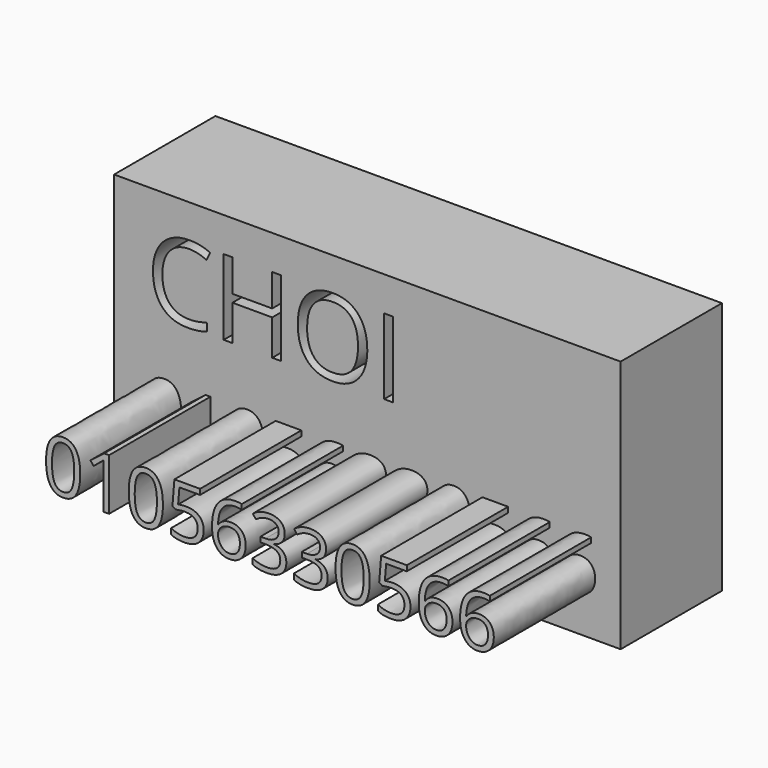
from build123d import *

# Parameters (mm, degrees)
F0_W         = 20
F0_H         = 10
F1_DEPTH     = 5
F2_TEXT_SIZE = 4.1780911346
F3_DEPTH     = 25
F4_TEXT_SIZE = 2.8558414973
F5_DEPTH     = 5


# Not quite as in the source:
# - Text() gives the source's letters only with a copy of the font that has no kerning and outlines rounded to 1/6400 em; it was checked with that copy


with BuildPart() as f1:
    # F0 (on Front) → F1 (new body)
    with BuildSketch(Plane.XZ):
        with Locations((10, 5)):
            Rectangle(F0_W, F0_H)
    extrude(amount=F1_DEPTH)

    # F2 (on face) → F3 (cut)
    with BuildSketch(Plane.XZ.offset(5)):
        with Locations((1.2794679289, 5.6590529445)):
            Text('CHOI', F2_TEXT_SIZE, font='Open Sans', text_align=(TextAlign.LEFT, TextAlign.BOTTOM))
    extrude(amount=-F3_DEPTH, mode=Mode.SUBTRACT)

    # F4 (on face) → F5 (join)
    with BuildSketch(Plane.XZ.offset(5)):
        with Locations((1.1709355749, 1.4716046862)):
            Text('01056330566', F4_TEXT_SIZE, font='Open Sans', text_align=(TextAlign.LEFT, TextAlign.BOTTOM))
    extrude(amount=F5_DEPTH)


solid = f1.part
